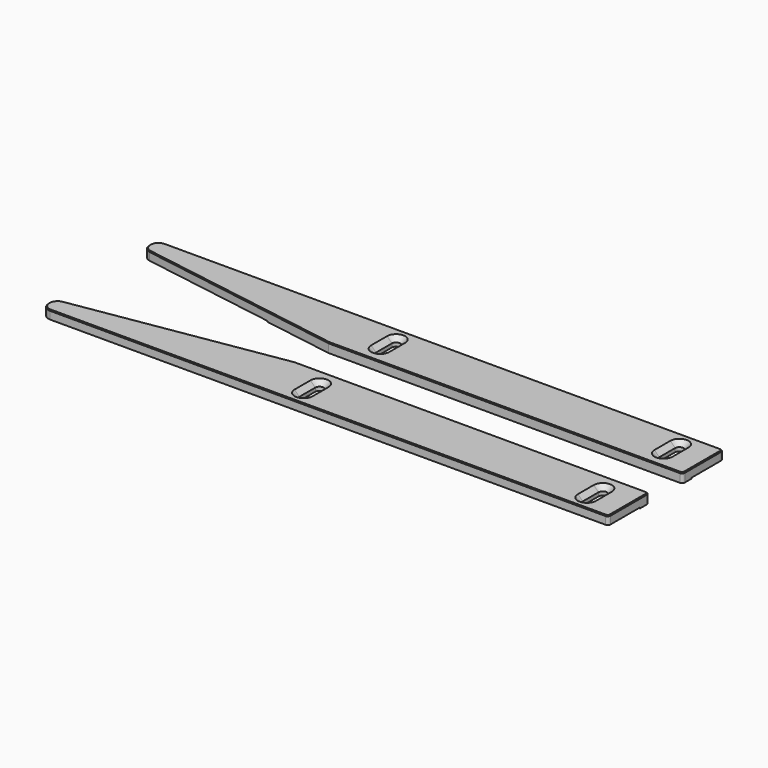
from build123d import *

# Parameters (mm, degrees)
F1_DEPTH    = 3
F3_DEPTH    = 0.3
F6_R        = 3
F6_2_R      = 3
F8_R        = 1
F8_2_R      = 1
F9_SIZE     = 0.3
F9_2_SIZE   = 0.3
F10_SIZE2   = 1.7
F10_SIZE    = 1.7
F10_2_SIZE2 = 1.7
F10_2_SIZE  = 1.7


# Not quite as in the source:
# - two fillets or chamfers of one size are made in one step
# - a feature names something its author has since deleted; it is built from what else it names


with BuildPart() as f1:
    # F0 (on Top) → F1 (new body)
    with BuildSketch(Plane.XY):
        Polygon((0, 5.8492044918), (0, 0), (200, 0), (200, 18), (75.0357434154, 18), align=None)
        with BuildLine():
            Line((89.974817574, 12), (89.974817574, 5))
            ThreePointArc((89.974817574, 5), (88.474817574, 3.5), (86.974817574, 5))
            Line((86.974817574, 5), (86.974817574, 12))
            ThreePointArc((86.974817574, 12), (88.474817574, 13.5), (89.974817574, 12))
        make_face(mode=Mode.SUBTRACT)
        with BuildLine():
            Line((189.974817574, 12), (189.974817574, 5))
            ThreePointArc((189.974817574, 5), (188.474817574, 3.5), (186.974817574, 5))
            Line((186.974817574, 5), (186.974817574, 12))
            ThreePointArc((186.974817574, 12), (188.474817574, 13.5), (189.974817574, 12))
        make_face(mode=Mode.SUBTRACT)
    extrude(amount=F1_DEPTH)

    # F2 (on face) → F3 (join)
    with BuildSketch(Plane(origin=(0, 0, 0), x_dir=(1, 0, 0), z_dir=(0, 0, -1))):
        Polygon((50.3342353158, -14), (75.0357434154, -18), (200, -18), (200, -14), align=None)
    extrude(amount=F3_DEPTH)


with BuildPart() as f5_1:
    # F5: instance of F1
    add(f1.part.mirror(Plane(origin=(100, 25.4, 1.5), x_dir=(1, 0, 0), z_dir=(0, -1, 0))))

    # F6#2
    f6_2_edges = [f5_1.edges().sort_by_distance(p)[0] for p in [
        (0, 44.950796, 1.5),
        (0, 50.8, 1.5),
    ]]
    fillet(f6_2_edges, radius=F6_2_R)

    # F8#2
    f8_2_edges = [f5_1.edges().sort_by_distance(p)[0] for p in [
        (200, 50.8, 1.5),
        (200, 32.8, 1.35),
    ]]
    fillet(f8_2_edges, radius=F8_2_R)

    # F9#2
    f9_2_edges = [f5_1.edges().sort_by_distance(p)[0] for p in [
        (137.017872, 32.8, 3),
        (200, 41.8, 3),
        (199.707107, 50.507107, 3),
        (101, 50.8, 3),
        (38.778095, 38.671325, 3),
        (0.87868, 49.92132, 3),
        (0.715415, 45.55968, 3),
        (0, 47.652037, 3),
        (199.707107, 33.092893, 3),
    ]]
    chamfer(f9_2_edges, length=F9_2_SIZE)

    # F10#2
    f10_2_edges = [f5_1.edges().sort_by_distance(p)[0] for p in [
        (189.974818, 42.3, 3),
        (188.474818, 37.3, 3),
        (186.974818, 42.3, 3),
        (188.474818, 47.3, 3),
        (88.474818, 47.3, 3),
        (89.974818, 42.3, 3),
        (88.474818, 37.3, 3),
        (86.974818, 42.3, 3),
    ]]
    chamfer(f10_2_edges, length=F10_2_SIZE, length2=F10_2_SIZE2)


with BuildPart() as f1_1:
    add(f1.part)

    # F6
    f6_edges = [f1_1.edges().sort_by_distance(p)[0] for p in [
        (0, 5.849204, 1.5),
        (0, 0, 1.5),
    ]]
    fillet(f6_edges, radius=F6_R)

    # F8
    f8_edges = [f1_1.edges().sort_by_distance(p)[0] for p in [
        (200, 0, 1.5),
        (200, 18, 1.35),
    ]]
    fillet(f8_edges, radius=F8_R)

    # F9
    f9_edges = [f1_1.edges().sort_by_distance(p)[0] for p in [
        (137.017872, 18, 3),
        (200, 9, 3),
        (199.707107, 0.292893, 3),
        (101, 0, 3),
        (38.778095, 12.128675, 3),
        (0.87868, 0.87868, 3),
        (0.715415, 5.24032, 3),
        (0, 3.147963, 3),
        (199.707107, 17.707107, 3),
    ]]
    chamfer(f9_edges, length=F9_SIZE)

    # F10
    f10_edges = [f1_1.edges().sort_by_distance(p)[0] for p in [
        (89.974818, 8.5, 3),
        (88.474818, 13.5, 3),
        (86.974818, 8.5, 3),
        (88.474818, 3.5, 3),
        (188.474818, 13.5, 3),
        (189.974818, 8.5, 3),
        (188.474818, 3.5, 3),
        (186.974818, 8.5, 3),
    ]]
    chamfer(f10_edges, length=F10_SIZE, length2=F10_SIZE2)


solid = Compound([f5_1.part, f1_1.part])
